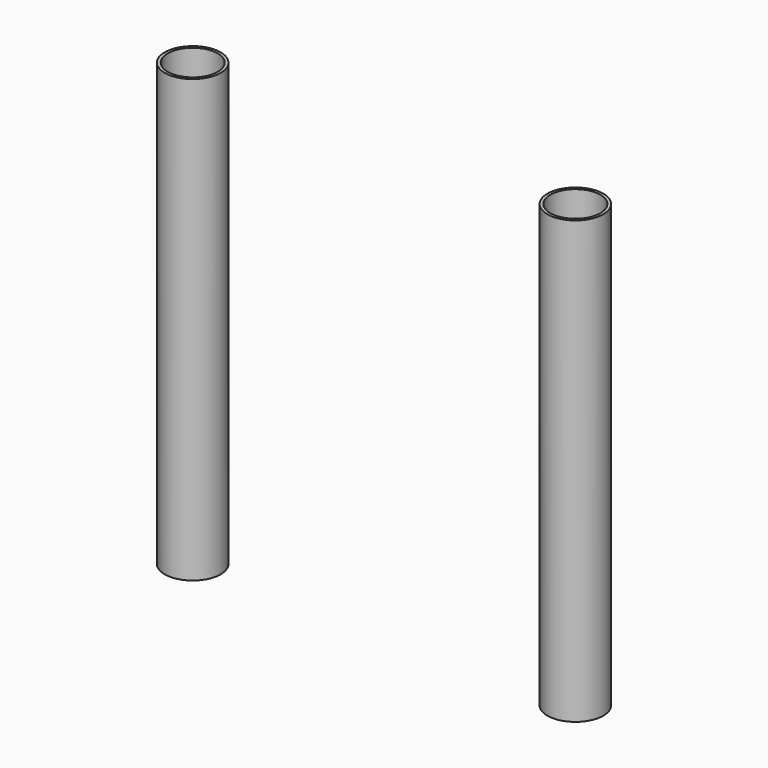
from build123d import *

# Parameters (mm, degrees)
F0_R     = 75
F0_R_2   = 9.5
F0_R_3   = 55
F1_DEPTH = 150
F2_R     = 75
F3_DEPTH = 5
F4_R     = 9.5
F4_R_2   = 8.5
F6_DEPTH = 150
F4_R_3   = 4.5949512094


# Not quite as in the source:
# - the program builds the solid bodies; features that only make, move or delete a surface that nothing else refers to are left out


with BuildPart() as f1:
    # F0 (on Top) → F1 (new body)
    with BuildSketch(Plane.XY):
        Circle(F0_R)
        with Locations((-64.9861544371, 0)):
            Circle(F0_R_2, mode=Mode.SUBTRACT)
        Circle(F0_R_3, mode=Mode.SUBTRACT)
        with Locations((65.034866333, 0)):
            Circle(F0_R_2, mode=Mode.SUBTRACT)
    extrude(amount=F1_DEPTH)

    # F2 (on face) → F3 (join)
    with BuildSketch(Plane(origin=(0, 0, 0), x_dir=(1, 0, 0), z_dir=(0, 0, -1))):
        Circle(F2_R)
    extrude(amount=F3_DEPTH)


with BuildPart() as f6:
    # F4 (on face) → F6 (new body)
    with BuildSketch(Plane.XY.offset(150)):
        with Locations((65.034866333, 0)):
            Circle(F4_R)
        with Locations((65.034866333, 0)):
            Circle(F4_R_2, mode=Mode.SUBTRACT)
    extrude(amount=F6_DEPTH)


with BuildPart() as f6b:
    # F4 (on face) → F6, piece 2 (new body)
    with BuildSketch(Plane.XY.offset(150)):
        with Locations((-64.9861544371, 0)):
            Circle(F4_R)
        with Locations((-64.9861544371, 0)):
            Circle(F4_R_2, mode=Mode.SUBTRACT)
    extrude(amount=F6_DEPTH)


with BuildPart() as f6c:
    # F4 (on face) → F6, piece 3 (new body)
    with BuildSketch(Plane.XY.offset(150)):
        with Locations((-6.2923626974, 0)):
            Circle(F4_R_3)
    extrude(amount=F6_DEPTH)


solid = Compound([f6.part, f6b.part])
